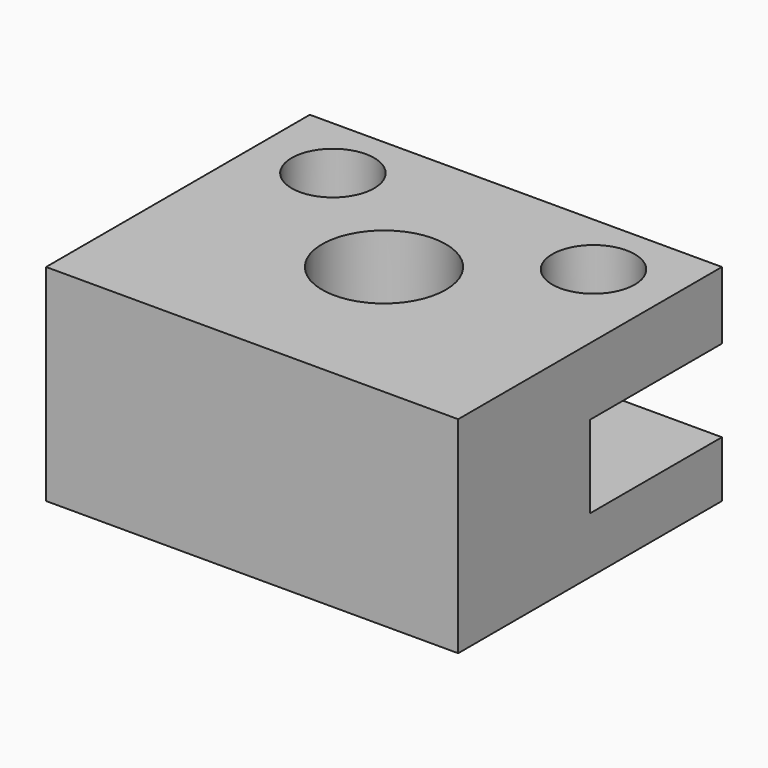
from build123d import *

# Parameters (mm, degrees)
F0_W     = 100
F0_H     = 80
F0_R     = 15
F1_DEPTH = 50
F3_W     = 122.5489005446
F3_H     = 20
F4_DEPTH = 40
F5_R     = 10
F6_DEPTH = 16.3678393885


# Not quite as in the source:
# - a pattern or mirror of a feature is missing from the dataset's text; its kind, count and spacing are read off the source's solid


with BuildPart() as f1:
    # F0 (on Top) → F1 (new body)
    with BuildSketch(Plane.XY):
        Rectangle(F0_W, F0_H)
        Circle(F0_R, mode=Mode.SUBTRACT)
    extrude(amount=F1_DEPTH)

    # F3 (on offset) → F4 (cut)
    with BuildSketch(Plane.XZ.offset(-40)):
        with Locations((0.9837634861, 23.6321606115)):
            Rectangle(F3_W, F3_H)
    extrude(amount=F4_DEPTH, mode=Mode.SUBTRACT)

    # F5 (on face) → F6 (cut, through all)
    with BuildSketch(Plane.XY.offset(50)):
        with Locations((31.620990485, 24.0319501609)):
            Circle(F5_R)
    f6 = extrude(amount=-F6_DEPTH, mode=Mode.SUBTRACT)

    # F6_copies: F6 across plane
    add(f6.mirror(Plane(origin=(0, 0, 0), x_dir=(0, 0, -1), z_dir=(-1, 0, 0))), mode=Mode.SUBTRACT)


solid = f1.part
